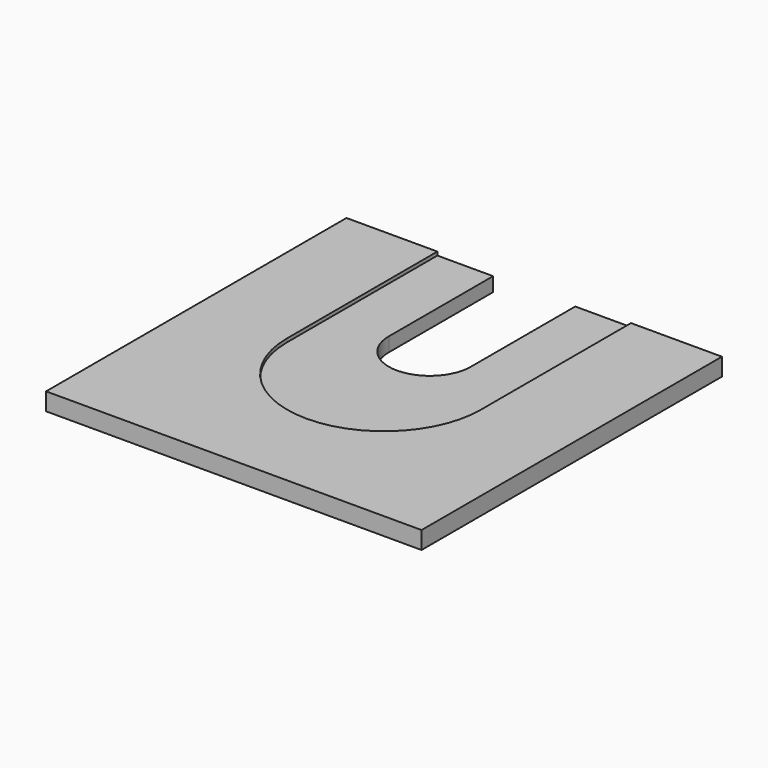
from build123d import *

# Parameters (mm, degrees)
F1_DEPTH = 9.525
F2_DEPTH = 7.62


# Not quite as in the source:
# - a feature names something its author has since deleted; it is built from what else it names


with BuildPart() as f1:
    # F0 (on Top) → F1 (new body)
    with BuildSketch(Plane.XY):
        with BuildLine():
            Line((-101.6, 101.6), (-101.6, -101.6))
            Line((-101.6, -101.6), (101.6, -101.6))
            Line((101.6, -101.6), (101.6, 101.6))
            Line((101.6, 101.6), (52.3875, 101.6))
            Line((52.3875, 101.6), (52.3875, 0))
            ThreePointArc((52.3875, 0), (0, -52.3875), (-52.3875, 0))
            Line((-52.3875, 0), (-52.3875, 101.6))
            Line((-52.3875, 101.6), (-101.6, 101.6))
        make_face()
    extrude(amount=F1_DEPTH)

    # F0 (on Top) → F2 (join)
    with BuildSketch(Plane.XY):
        with BuildLine():
            Line((-22.225, 101.6), (-52.3875, 101.6))
            Line((-52.3875, 101.6), (-52.3875, 0))
            ThreePointArc((-52.3875, 0), (-44.2083835022, 28.1081657953), (-22.225, 47.439430132))
            Line((-22.225, 47.439430132), (-22.225, 101.6))
        make_face()
        with BuildLine():
            Line((52.3875, 0), (52.3875, 101.6))
            Line((52.3875, 101.6), (22.225, 101.6))
            Line((22.225, 101.6), (22.225, 47.439430132))
            ThreePointArc((22.225, 47.439430132), (44.2083835022, 28.1081657953), (52.3875, 0))
        make_face()
        with BuildLine():
            ThreePointArc((-22.225, 47.439430132), (-44.2083835022, 28.1081657953), (-52.3875, 0))
            ThreePointArc((-52.3875, 0), (0, -52.3875), (52.3875, 0))
            ThreePointArc((52.3875, 0), (44.2083835022, 28.1081657953), (22.225, 47.439430132))
            Line((22.225, 47.439430132), (22.225, 31))
            ThreePointArc((22.225, 31), (0, 8.775), (-22.225, 31))
            Line((-22.225, 31), (-22.225, 47.439430132))
        make_face()
    extrude(amount=F2_DEPTH)


solid = f1.part
